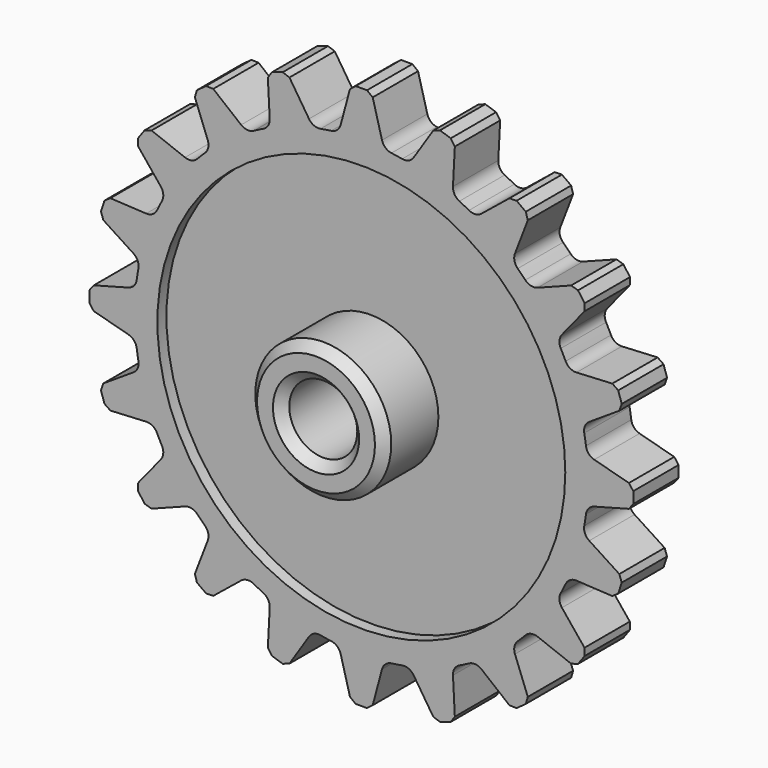
from build123d import *

# Parameters (mm, degrees)
F0_R            = 100
F1_DEPTH        = 25
F3_DEPTH        = 25
F3_COPIES_COUNT = 20
F4_SIZE         = 2
F5_R            = 5
F6_R            = 90
F7_DEPTH        = 5
F8_R            = 30
F9_DEPTH        = 30
F10_R           = 15
F11_DEPTH       = 50.001
F12_SIZE        = 4


# Not quite as in the source:
# - a pattern or mirror of a feature is missing from the dataset's text; its kind, count and spacing are read off the source's solid


with BuildPart() as f1:
    # F0 (on Front) → F1 (new body)
    with BuildSketch(Plane.XZ):
        Circle(F0_R)
    extrude(amount=F1_DEPTH)

    # F2 (on Front) → F3 (join)
    with BuildSketch(Plane.XZ):
        Polygon((-4.5, 120), (-9.9931095726, 99.4994359837), (9.9931095726, 99.4994359837), (4.5, 120), align=None)
    f3 = extrude(amount=F3_DEPTH)

    # F3_copies: F3 ×20 about axis
    f3_copies_axis = Axis((0, 0, 0), (0, 1, 0))
    for i in range(1, F3_COPIES_COUNT):
        add(f3.rotate(f3_copies_axis, i * 360 / F3_COPIES_COUNT))

    # F4
    f4_edges = [f1.edges().sort_by_distance(p)[0] for p in [
        (-4.5, -12.5, 120),
        (4.5, -12.5, 120),
        (-32.802285, -12.5, 115.517358),
        (115.517358, -12.5, 32.802285),
        (120, -12.5, 4.5),
        (120, -12.5, -4.5),
        (115.517358, -12.5, -32.802285),
        (112.736205, -12.5, -41.361794),
        (99.727073, -12.5, -66.893654),
        (94.437006, -12.5, -74.174807),
        (74.174807, -12.5, -94.437006),
        (66.893654, -12.5, -99.727073),
        (41.361794, -12.5, -112.736205),
        (32.802285, -12.5, -115.517358),
        (4.5, -12.5, -120),
        (-4.5, -12.5, -120),
        (-32.802285, -12.5, -115.517358),
        (-41.361794, -12.5, -112.736205),
        (-66.893654, -12.5, -99.727073),
        (-74.174807, -12.5, -94.437006),
        (-94.437006, -12.5, -74.174807),
        (-99.727073, -12.5, -66.893654),
        (-112.736205, -12.5, -41.361794),
        (-115.517358, -12.5, -32.802285),
        (-120, -12.5, -4.5),
        (-120, -12.5, 4.5),
        (-115.517358, -12.5, 32.802285),
        (-112.736205, -12.5, 41.361794),
        (-99.727073, -12.5, 66.893654),
        (-94.437006, -12.5, 74.174807),
        (-74.174807, -12.5, 94.437006),
        (-66.893654, -12.5, 99.727073),
        (32.802285, -12.5, 115.517358),
        (41.361794, -12.5, 112.736205),
        (66.893654, -12.5, 99.727073),
        (74.174807, -12.5, 94.437006),
        (94.437006, -12.5, 74.174807),
        (99.727073, -12.5, 66.893654),
        (112.736205, -12.5, 41.361794),
        (-41.361794, -12.5, 112.736205),
    ]]
    chamfer(f4_edges, length=F4_SIZE)

    # F5
    f5_edges = [f1.edges().sort_by_distance(p)[0] for p in [
        (9.99311, -12.5, 99.499436),
        (-9.99311, -12.5, 99.499436),
        (97.717628, -12.5, 21.243005),
        (99.499436, -12.5, 9.99311),
        (91.541546, -12.5, 40.251029),
        (86.370537, -12.5, 50.399706),
        (99.499436, -12.5, -9.99311),
        (97.717628, -12.5, -21.243005),
        (74.622932, -12.5, 66.568897),
        (66.568897, -12.5, 74.622932),
        (91.541546, -12.5, -40.251029),
        (86.370537, -12.5, -50.399706),
        (50.399706, -12.5, 86.370537),
        (40.251029, -12.5, 91.541546),
        (74.622932, -12.5, -66.568897),
        (66.568897, -12.5, -74.622932),
        (21.243005, -12.5, 97.717628),
        (50.399706, -12.5, -86.370537),
        (40.251029, -12.5, -91.541546),
        (-21.243005, -12.5, 97.717628),
        (21.243005, -12.5, -97.717628),
        (9.99311, -12.5, -99.499436),
        (-40.251029, -12.5, 91.541546),
        (-50.399706, -12.5, 86.370537),
        (-9.99311, -12.5, -99.499436),
        (-21.243005, -12.5, -97.717628),
        (-66.568897, -12.5, 74.622932),
        (-74.622932, -12.5, 66.568897),
        (-40.251029, -12.5, -91.541546),
        (-50.399706, -12.5, -86.370537),
        (-86.370537, -12.5, 50.399706),
        (-91.541546, -12.5, 40.251029),
        (-66.568897, -12.5, -74.622932),
        (-74.622932, -12.5, -66.568897),
        (-97.717628, -12.5, 21.243005),
        (-99.499436, -12.5, 9.99311),
        (-86.370537, -12.5, -50.399706),
        (-91.541546, -12.5, -40.251029),
        (-99.499436, -12.5, -9.99311),
        (-97.717628, -12.5, -21.243005),
    ]]
    fillet(f5_edges, radius=F5_R)

    # F6 (on face) → F7 (cut)
    with BuildSketch(Plane.XZ.offset(25)):
        Circle(F6_R)
    extrude(amount=-F7_DEPTH, mode=Mode.SUBTRACT)

    # F8 (on face) → F9 (join)
    with BuildSketch(Plane.XZ.offset(20)):
        Circle(F8_R)
    extrude(amount=F9_DEPTH)

    # F10 (on face) → F11 (cut, through all)
    with BuildSketch(Plane.XZ.offset(50)):
        Circle(F10_R)
    extrude(amount=-F11_DEPTH, mode=Mode.SUBTRACT)

    # F12
    f12_edges = [f1.edges().sort_by_distance(p)[0] for p in [
        (-30, -50, 0),
        (-15, -50, 0),
    ]]
    chamfer(f12_edges, length=F12_SIZE)


solid = f1.part
